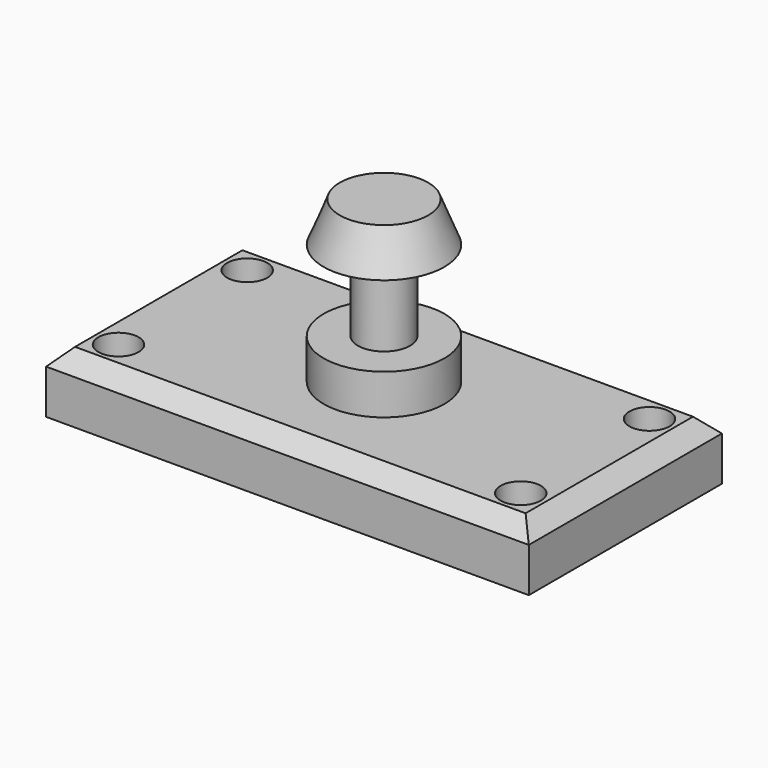
from build123d import *

# Parameters (mm, degrees)
F0_W     = 152.4
F0_H     = 76.2
F1_DEPTH = 19.05
F2_R     = 6.35
F3_DEPTH = 19.051
F4_W     = 19.05
F4_H     = 50.8
F6_SIZE  = 5.08
F7_W     = 10.795
F7_H     = 25.4
F9_SIZE2 = 5.07999
F9_SIZE  = 12.69999


# Not quite as in the source:
# - a fillet or chamfer is up to 0.001 mm smaller than in the source, because OpenCascade refuses the exact size


with BuildPart() as f1:
    # F0 (on Top) → F1 (new body)
    with BuildSketch(Plane.XY):
        Rectangle(F0_W, F0_H)
    extrude(amount=F1_DEPTH)

    # F2 (on Top) → F3 (cut, through all)
    with BuildSketch(Plane.XY):
        with Locations((-63.5, 25.4)):
            Circle(F2_R)
        with Locations((63.5, -25.4)):
            Circle(F2_R)
        with Locations((63.5, 25.4)):
            Circle(F2_R)
        with Locations((-63.5, -25.4)):
            Circle(F2_R)
    extrude(amount=F3_DEPTH, mode=Mode.SUBTRACT)

    # F4 (on Front) → F5 (revolve)
    with BuildSketch(Plane.XZ):
        with Locations((9.525, 44.45)):
            Rectangle(F4_W, F4_H)
    revolve(axis=Axis((0, 0, 44.45), (0, 0, -1)))

    # F6
    f6_edges = [f1.edges().sort_by_distance(p)[0] for p in [
        (0, -38.1, 19.05),
        (-76.2, 0, 19.05),
        (0, 38.1, 19.05),
        (76.2, 0, 19.05),
    ]]
    chamfer(f6_edges, length=F6_SIZE)

    # F7 (on Front) → F8 (revolve, cut)
    with BuildSketch(Plane.XZ):
        with Locations((13.6525, 44.45)):
            Rectangle(F7_W, F7_H)
    revolve(axis=Axis((0, 0, 19.05), (0, 0, 1)), mode=Mode.SUBTRACT)

    # F9 (size 12.7 and 5.08 in the source; OpenCascade refuses exactly that, so slightly less here)
    f9_edges = [f1.edges().sort_by_distance(p)[0] for p in [
        (-19.05, 0, 69.85),
    ]]
    f9_side = f1.faces().sort_by_distance((-19.05, 0, 63.5))[0]
    chamfer(f9_edges, length=F9_SIZE, length2=F9_SIZE2, reference=f9_side)


solid = f1.part
